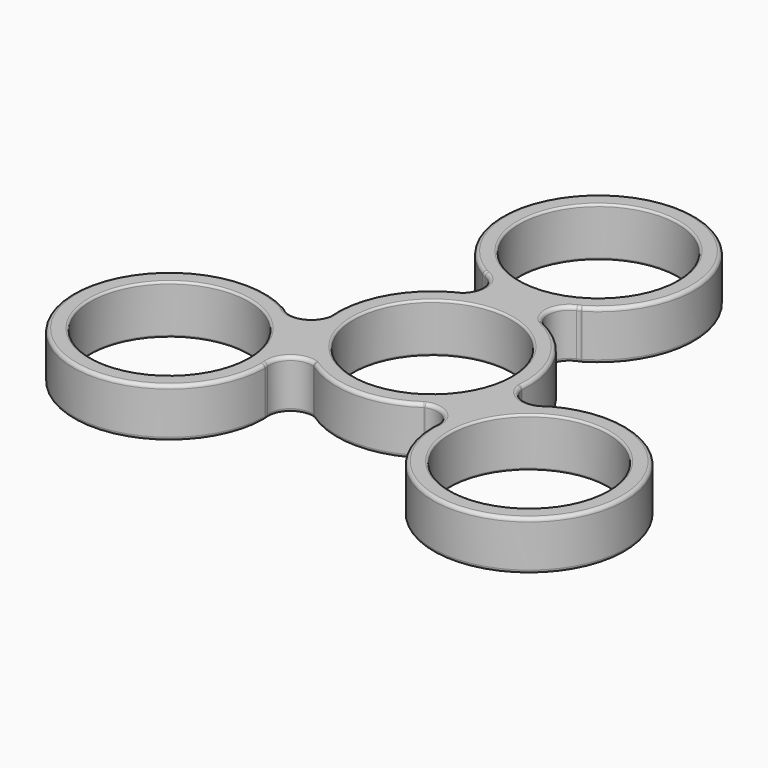
from build123d import *

# Parameters (mm, degrees)
F0_R     = 11.2
F1_DEPTH = 7
F3_COUNT = 3
F4_R     = 0.5
F5_R     = 0.3


# Not quite as in the source:
# - a feature names something its author has since deleted; it is built from what else it names


with BuildPart() as f1:
    # F0 (on Top) → F1 (new body)
    with BuildSketch(Plane.XY):
        with BuildLine():
            Line((6.5006651649, 17.5112300987), (7, 17.7233281442))
            ThreePointArc((7, 17.7233281442), (0, 43.2), (-7, 17.7233281442))
            Line((-7, 17.7233281442), (-6.5006651649, 17.5112300987))
            ThreePointArc((-6.5006651649, 17.5112300987), (-4.6735284742, 14.75), (-6.5006651649, 11.9887699013))
            Line((-6.5006651649, 11.9887699013), (-7, 11.7766718558))
            ThreePointArc((-7, 11.7766718558), (0, -13.7), (7, 11.7766718558))
            Line((7, 11.7766718558), (6.5006651649, 11.9887699013))
            ThreePointArc((6.5006651649, 11.9887699013), (4.6735284742, 14.75), (6.5006651649, 17.5112300987))
        make_face()
        Circle(F0_R, mode=Mode.SUBTRACT)
        with Locations((0, 29.5)):
            Circle(F0_R, mode=Mode.SUBTRACT)
    extrude(amount=F1_DEPTH)

    # F3: F1 ×3 about axis
    f3_axis = Axis((0, 0, 1.5517235734), (0, 0, 1))


with BuildPart() as f1_1:
    add(f1.part)
    for i in range(1, F3_COUNT):
        add(f1.part.rotate(f3_axis, i * 360 / F3_COUNT))

    # F4
    f4_edges = [f1_1.edges().sort_by_distance(p)[0] for p in [
        (0, -13.7, 0),
        (-7.861518, -11.219917, 3.5),
        (0, -13.7, 7),
        (7.861518, -11.219917, 3.5),
        (11.864548, 6.85, 0),
        (13.647492, -1.198316, 3.5),
        (11.864548, 6.85, 7),
        (5.785974, 12.418233, 3.5),
        (-5.785974, 12.418233, 3.5),
        (-11.864548, 6.85, 7),
        (-13.647492, -1.198316, 3.5),
        (-11.864548, 6.85, 0),
        (-18.848852, -2.799486, 3.5),
        (-11.848852, -14.923842, 3.5),
        (-37.412297, -21.6, 0),
        (-37.412297, -21.6, 7),
        (-10.783602, -11.656053, 0),
        (-10.783602, -11.656053, 7),
        (-11.914838, -14.385356, 3.5),
        (-15.486239, -3.510847, 0),
        (-18.415503, -3.125874, 3.5),
        (-15.486239, -3.510847, 7),
        (10.783602, -11.656053, 0),
        (11.914838, -14.385356, 3.5),
        (10.783602, -11.656053, 7),
        (11.848852, -14.923842, 3.5),
        (18.848852, -2.799486, 3.5),
        (37.412297, -21.6, 0),
        (37.412297, -21.6, 7),
        (15.486239, -3.510847, 0),
        (15.486239, -3.510847, 7),
        (18.415503, -3.125874, 3.5),
        (4.702637, 15.1669, 0),
        (6.500665, 17.51123, 3.5),
        (4.702637, 15.1669, 7),
        (7, 17.723328, 3.5),
        (-7, 17.723328, 3.5),
        (0, 43.2, 0),
        (0, 43.2, 7),
        (-4.702637, 15.1669, 0),
        (-4.702637, 15.1669, 7),
        (-6.500665, 17.51123, 3.5),
    ]]
    fillet(f4_edges, radius=F4_R)

    # F5
    f5_edges = [f1_1.edges().sort_by_distance(p)[0] for p in [
        (11.2, 29.5, 3.5),
        (-11.2, 29.5, 0),
        (-11.2, 29.5, 7),
        (-11.2, 0, 0),
        (11.2, 0, 3.5),
        (-11.2, 0, 7),
        (19.947749, -24.449485, 3.5),
        (31.147749, -5.050515, 0),
        (31.147749, -5.050515, 7),
        (-31.147749, -5.050515, 3.5),
        (-19.947749, -24.449485, 0),
        (-19.947749, -24.449485, 7),
    ]]
    fillet(f5_edges, radius=F5_R)


solid = f1_1.part
